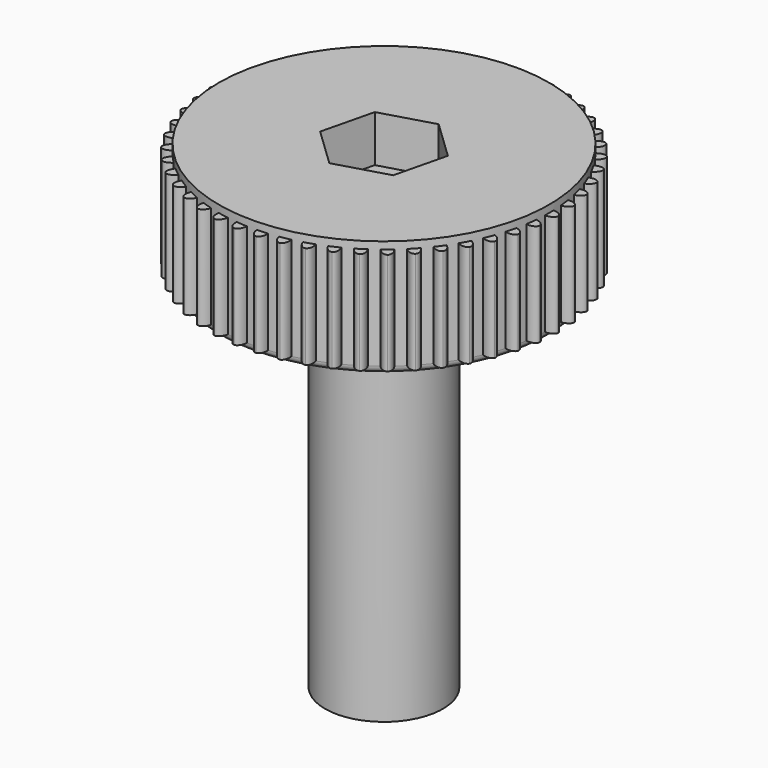
from build123d import *

# Parameters (mm, degrees)
F0_W            = 0.7
F0_H            = 12
F2_R            = 1
F5_DEPTH        = 14.3
F5_COPIES_COUNT = 50
F6_R            = 3.525
F7_DEPTH        = 6.5


# Not quite as in the source:
# - a pattern or mirror of a feature is missing from the dataset's text; its kind, count and spacing are read off the source's solid
# - a feature names something its author has since deleted; it is built from what else it names


with BuildPart() as f1:
    # F0 (on Front) → F1 (revolve)
    with BuildSketch(Plane.XZ):
        Polygon((-7.5, -20), (-7.5, 7.0330877347), (-7.5, 17.3905188113), (-7.5, 27), (-3.525, 27), (-3.525, 28.3), (-3.525, 34.6), (-23, 34.6), (-23, 28.3), (-23, 18.3), (-8.2, 18.3), (-8.2, -20), align=None)
        with Locations((-7.85, -26)):
            Rectangle(F0_W, F0_H)
    revolve(axis=Axis((0, 0, 15.8405188113), (0, 0, -1)))

    # F2
    f2_edges = [f1.edges().sort_by_distance(p)[0] for p in [
        (8.2, 0, 18.3),
        (23, 0, 18.3),
    ]]
    fillet(f2_edges, radius=F2_R)

    # F4 (on offset) → F5 (join)
    with BuildSketch(Plane.XY.offset(33.6)):
        with BuildLine():
            add(Edge.make_bspline(
                [(24.25, 0), (24.25, 1.2990381057), (22.375, 0.6495190528), (20.5, 0), (22.375, -0.6495190528), (24.25, -1.2990381057), (24.25, 0)],
                knots=[0, 0, 0, 2.0943951024, 2.0943951024, 4.1887902048, 4.1887902048, 6.2831853072, 6.2831853072, 6.2831853072], degree=2, weights=[1, 0.5, 1, 0.5, 1, 0.5, 1]))
        make_face()
    f5 = extrude(amount=-F5_DEPTH)

    # F5_copies: F5 ×50 about axis
    f5_copies_axis = Axis((0, 0, 0), (0, 0, 1))
    for i in range(1, F5_COPIES_COUNT):
        add(f5.rotate(f5_copies_axis, i * 360 / F5_COPIES_COUNT))

    # F6 (on face) → F7 (cut)
    with BuildSketch(Plane.XY.offset(34.6)):
        Polygon((-7.2035379805, -2.107693976), (-1.7764524637, -7.2922938762), (5.4270855169, -5.1845999003), (7.2035379805, 2.107693976), (1.7764524637, 7.2922938762), (-5.4270855169, 5.1845999003), align=None)
        Circle(F6_R, mode=Mode.SUBTRACT)
    extrude(amount=-F7_DEPTH, mode=Mode.SUBTRACT)


solid = f1.part
